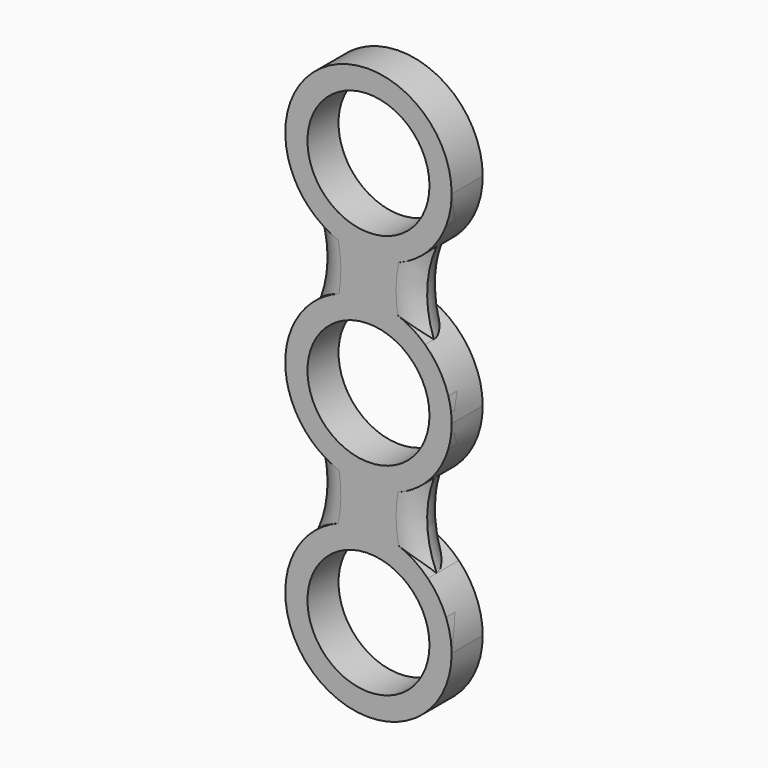
from build123d import *

# Parameters (mm, degrees)
F0_R         = 11.176
F1_DEPTH     = 7.112
F2_T4_ANGLE  = 116.1586222886
F2_S5_R      = 15.24
F2_T6_DEPTH  = 30
F2_S7_R      = 15.24
F2_T8_DEPTH  = 30
F2_T12_ANGLE = 116.1586222886
F2_S13_R     = 15.24
F2_T14_DEPTH = 30
F2_S15_R     = 15.24
F2_T16_DEPTH = 30
F3_R         = 5.08
F4_T4_ANGLE  = 101.759749901
F4_S5_R      = 15.24
F4_T6_DEPTH  = 23
F4_S7_R      = 15.24
F4_T8_DEPTH  = 23
F4_T12_ANGLE = 101.7597499017
F4_S13_R     = 15.24
F4_T14_DEPTH = 27
F4_S15_R     = 15.24
F4_T16_DEPTH = 27
F4_T20_ANGLE = 101.7597499014
F4_S21_R     = 15.24
F4_T22_DEPTH = 27
F4_S23_R     = 15.24
F4_T24_DEPTH = 27
F4_T28_ANGLE = 101.7597499014
F4_S29_R     = 15.24
F4_T30_DEPTH = 27
F4_S31_R     = 15.24
F4_T32_DEPTH = 27


# Not quite as in the source:
# - a fillet or chamfer that OpenCascade refuses, or shapes differently, is made with other operations: its cross-section is extruded or revolved along the edge and cut away or added


with BuildPart() as f1:
    # F0 (on Front) → F1 (new body)
    with BuildSketch(Plane.XZ):
        with BuildLine():
            ThreePointArc((10.3608125449, -11.1763662883), (13.9670394713, -6.0974919769), (15.24, 0))
            ThreePointArc((15.24, 0), (13.9670394713, 6.0974919769), (10.3608125449, 11.1763662883))
            ThreePointArc((10.3608125449, 11.1763662883), (0, 15.24), (-10.3608125449, 11.1763662883))
            ThreePointArc((-10.3608125449, 11.1763662883), (-15.24, 0), (-10.3608125449, -11.1763662883))
            ThreePointArc((-10.3608125449, -11.1763662883), (0, -15.24), (10.3608125449, -11.1763662883))
        make_face()
        Circle(F0_R, mode=Mode.SUBTRACT)
        with BuildLine():
            ThreePointArc((-10.3608125449, 11.1763662883), (0, 15.24), (10.3608125449, 11.1763662883))
            ThreePointArc((10.3608125449, 11.1763662883), (9.1357508424, 18.8221602784), (10.8748760535, 26.3676480303))
            ThreePointArc((10.8748760535, 26.3676480303), (0, 21.8044767177), (-10.8748760535, 26.3676480303))
            ThreePointArc((-10.8748760535, 26.3676480303), (-9.1357508424, 18.8221602784), (-10.3608125449, 11.1763662883))
        make_face()
        with BuildLine():
            ThreePointArc((10.8748760535, -26.3676480303), (9.1357508424, -18.8221602784), (10.3608125449, -11.1763662883))
            ThreePointArc((10.3608125449, -11.1763662883), (0, -15.24), (-10.3608125449, -11.1763662883))
            ThreePointArc((-10.3608125449, -11.1763662883), (-9.1357508424, -18.8221602784), (-10.8748760535, -26.3676480303))
            ThreePointArc((-10.8748760535, -26.3676480303), (0, -21.8044767177), (10.8748760535, -26.3676480303))
        make_face()
        with BuildLine():
            ThreePointArc((-10.8748760535, 26.3676480303), (0, 21.8044767177), (10.8748760535, 26.3676480303))
            ThreePointArc((10.8748760535, 26.3676480303), (14.1065713598, 31.2771337877), (15.24, 37.0444767177))
            ThreePointArc((15.24, 37.0444767177), (-5.76734293, 51.1510480775), (-10.8748760535, 26.3676480303))
        make_face()
        with Locations((0, 37.0444767177)):
            Circle(F0_R, mode=Mode.SUBTRACT)
        with BuildLine():
            ThreePointArc((15.24, -37.0444767177), (14.1065713598, -31.2771337877), (10.8748760535, -26.3676480303))
            ThreePointArc((10.8748760535, -26.3676480303), (0, -21.8044767177), (-10.8748760535, -26.3676480303))
            ThreePointArc((-10.8748760535, -26.3676480303), (-5.76734293, -51.1510480775), (15.24, -37.0444767177))
        make_face()
        with Locations((0, -37.0444767177)):
            Circle(F0_R, mode=Mode.SUBTRACT)
    extrude(amount=F1_DEPTH)

    # F2: fillet of radius 5.08 on 2 edges, made by hand


with BuildPart() as f2_tool2:
    # F2_s3 → F2_t4 (revolve)
    with BuildSketch(Plane(origin=(29.8644460088, 0, -17.2301380427), x_dir=(0, 1, 0), z_dir=(0.8661774261, 0, -0.4997365971))):
        with BuildLine():
            ThreePointArc((-5.08, -21.2648569422), (-1.4878975516, -22.7527544938), (0, -26.3448569422))
            Line((0, -26.3448569422), (0, -21.2648569422))
            Line((0, -21.2648569422), (-5.08, -21.2648569422))
        make_face()
    revolve(axis=Axis((29.340401561, 0, -18.1384474874), (0, 1, 0)), revolution_arc=F2_T4_ANGLE)

    # F2_s5 → F2_t6 (cut, symmetric)
    with BuildSketch(Plane.XZ.offset(2.5)):
        with Locations((0, -37.0444767177)):
            Circle(F2_S5_R)
    extrude(amount=F2_T6_DEPTH, both=True, mode=Mode.SUBTRACT)

    # F2_s7 → F2_t8 (cut, symmetric)
    with BuildSketch(Plane.XZ.offset(2.5)):
        Circle(F2_S7_R)
    extrude(amount=F2_T8_DEPTH, both=True, mode=Mode.SUBTRACT)


with BuildPart() as f1_1:
    add(f1.part)

    # F2_t1: cut F2_tool2
    add(f2_tool2.part, mode=Mode.SUBTRACT)


with BuildPart() as f2_tool10:
    # F2_s11 → F2_t12 (revolve)
    with BuildSketch(Plane(origin=(-11.8407369211, 0, 7.9442927806), x_dir=(0, 1, 0), z_dir=(-0.8304131044, 0, 0.5571481635))):
        with BuildLine():
            ThreePointArc((-5.08, 11.1931397161), (-1.4878975516, 9.7052421646), (0, 6.1131397161))
            Line((0, 6.1131397161), (0, 11.1931397161))
            Line((0, 11.1931397161), (-5.08, 11.1931397161))
        make_face()
    revolve(axis=Axis((-29.340401561, 0, -18.1384474874), (0, 1, 0)), revolution_arc=F2_T12_ANGLE)

    # F2_s13 → F2_t14 (cut, symmetric)
    with BuildSketch(Plane.XZ.offset(4.3)):
        Circle(F2_S13_R)
    extrude(amount=F2_T14_DEPTH, both=True, mode=Mode.SUBTRACT)

    # F2_s15 → F2_t16 (cut, symmetric)
    with BuildSketch(Plane.XZ.offset(4.3)):
        with Locations((0, -37.0444767177)):
            Circle(F2_S15_R)
    extrude(amount=F2_T16_DEPTH, both=True, mode=Mode.SUBTRACT)


with BuildPart() as f1_2:
    add(f1_1.part)

    # F2_t9: cut F2_tool10
    add(f2_tool10.part, mode=Mode.SUBTRACT)

    # F3#2 (call 1 of 2: OpenCascade refuses the feature's edges together)
    f3_2_edges = [f1_2.edges().sort_by_distance(p)[0] for p in [
        (-9.135751, 0, 18.82216),
    ]]
    fillet(f3_2_edges, radius=F3_R)

    # F3 (call 2 of 2)
    f3_edges = [f1_2.edges().sort_by_distance(p)[0] for p in [
        (9.135751, 0, 18.82216),
    ]]
    fillet(f3_edges, radius=F3_R)

    # F4: fillet of radius 5.08 on 4 edges, made by hand


with BuildPart() as f4_tool2:
    # F4_s3 → F4_t4 (revolve)
    with BuildSketch(Plane(origin=(27.3577839274, 0, -20.7521533482), x_dir=(0, 1, 0), z_dir=(0.7967197018, 0, -0.6043490025))):
        with BuildLine():
            ThreePointArc((-7.112, -20.9996316731), (-6.5756901303, -18.727786608), (-5.08, -16.9356316731))
            Line((-5.08, -16.9356316731), (-7.112, -16.9356316732))
            Line((-7.112, -16.9356316732), (-7.112, -20.9996316731))
        make_face()
    revolve(axis=Axis((29.340401561, -7.112, -18.1384474874), (0, 1, 0)), revolution_arc=F4_T4_ANGLE)

    # F4_s5 → F4_t6 (cut, symmetric)
    with BuildSketch(Plane.XZ.offset(4.6)):
        Circle(F4_S5_R)
    extrude(amount=F4_T6_DEPTH, both=True, mode=Mode.SUBTRACT)

    # F4_s7 → F4_t8 (cut, symmetric)
    with BuildSketch(Plane.XZ.offset(4.6)):
        with Locations((0, -37.0444767177)):
            Circle(F4_S7_R)
    extrude(amount=F4_T8_DEPTH, both=True, mode=Mode.SUBTRACT)


with BuildPart() as f1_3:
    add(f1_2.part)

    # F4_t1: cut F4_tool2
    add(f4_tool2.part, mode=Mode.SUBTRACT)


with BuildPart() as f4_tool10:
    # F4_s11 → F4_t12 (revolve)
    with BuildSketch(Plane(origin=(-7.6988506956, 0, 6.7062600285), x_dir=(0, 1, 0), z_dir=(-0.7540423315, 0, 0.6568258234))):
        with BuildLine():
            ThreePointArc((-7.112, 8.6684750316), (-6.5756901303, 10.9403200968), (-5.08, 12.7324750316))
            Line((-5.08, 12.7324750316), (-7.112, 12.7324750316))
            Line((-7.112, 12.7324750316), (-7.112, 8.6684750316))
        make_face()
    revolve(axis=Axis((-29.340401561, -7.112, -18.1384474874), (0, 1, 0)), revolution_arc=F4_T12_ANGLE)

    # F4_s13 → F4_t14 (cut, symmetric)
    with BuildSketch(Plane.XZ.offset(4.6)):
        with Locations((0, -37.0444767177)):
            Circle(F4_S13_R)
    extrude(amount=F4_T14_DEPTH, both=True, mode=Mode.SUBTRACT)

    # F4_s15 → F4_t16 (cut, symmetric)
    with BuildSketch(Plane.XZ.offset(4.6)):
        Circle(F4_S15_R)
    extrude(amount=F4_T16_DEPTH, both=True, mode=Mode.SUBTRACT)


with BuildPart() as f1_4:
    add(f1_3.part)

    # F4_t9: cut F4_tool10
    add(f4_tool10.part, mode=Mode.SUBTRACT)


with BuildPart() as f4_tool18:
    # F4_s19 → F4_t20 (revolve)
    with BuildSketch(Plane(origin=(-27.3577839275, 0, 20.7521533481), x_dir=(0, 1, 0), z_dir=(-0.7967197018, 0, 0.6043490025))):
        with BuildLine():
            ThreePointArc((-7.112, -20.9996316733), (-6.5756901303, -18.7277866081), (-5.08, -16.9356316733))
            Line((-5.08, -16.9356316733), (-7.112, -16.9356316733))
            Line((-7.112, -16.9356316733), (-7.112, -20.9996316733))
        make_face()
    revolve(axis=Axis((-29.340401561, -7.112, 18.1384474874), (0, 1, 0)), revolution_arc=F4_T20_ANGLE)

    # F4_s21 → F4_t22 (cut, symmetric)
    with BuildSketch(Plane.XZ.offset(4.6)):
        with Locations((0, 37.0444767177)):
            Circle(F4_S21_R)
    extrude(amount=F4_T22_DEPTH, both=True, mode=Mode.SUBTRACT)

    # F4_s23 → F4_t24 (cut, symmetric)
    with BuildSketch(Plane.XZ.offset(4.6)):
        Circle(F4_S23_R)
    extrude(amount=F4_T24_DEPTH, both=True, mode=Mode.SUBTRACT)


with BuildPart() as f1_5:
    add(f1_4.part)

    # F4_t17: cut F4_tool18
    add(f4_tool18.part, mode=Mode.SUBTRACT)


with BuildPart() as f4_tool26:
    # F4_s27 → F4_t28 (revolve)
    with BuildSketch(Plane(origin=(7.6988506955, 0, -6.7062600285), x_dir=(0, 1, 0), z_dir=(0.7540423315, 0, -0.6568258234))):
        with BuildLine():
            ThreePointArc((-5.08, 12.7324750317), (-6.5756901303, 10.9403200968), (-7.112, 8.6684750317))
            Line((-7.112, 8.6684750317), (-7.112, 12.7324750317))
            Line((-7.112, 12.7324750317), (-5.08, 12.7324750317))
        make_face()
    revolve(axis=Axis((29.340401561, -7.112, 18.1384474874), (0, 1, 0)), revolution_arc=F4_T28_ANGLE)

    # F4_s29 → F4_t30 (cut, symmetric)
    with BuildSketch(Plane.XZ.offset(4.6)):
        Circle(F4_S29_R)
    extrude(amount=F4_T30_DEPTH, both=True, mode=Mode.SUBTRACT)

    # F4_s31 → F4_t32 (cut, symmetric)
    with BuildSketch(Plane.XZ.offset(4.6)):
        with Locations((0, 37.0444767177)):
            Circle(F4_S31_R)
    extrude(amount=F4_T32_DEPTH, both=True, mode=Mode.SUBTRACT)


with BuildPart() as f1_6:
    add(f1_5.part)

    # F4_t25: cut F4_tool26
    add(f4_tool26.part, mode=Mode.SUBTRACT)


solid = f1_6.part
